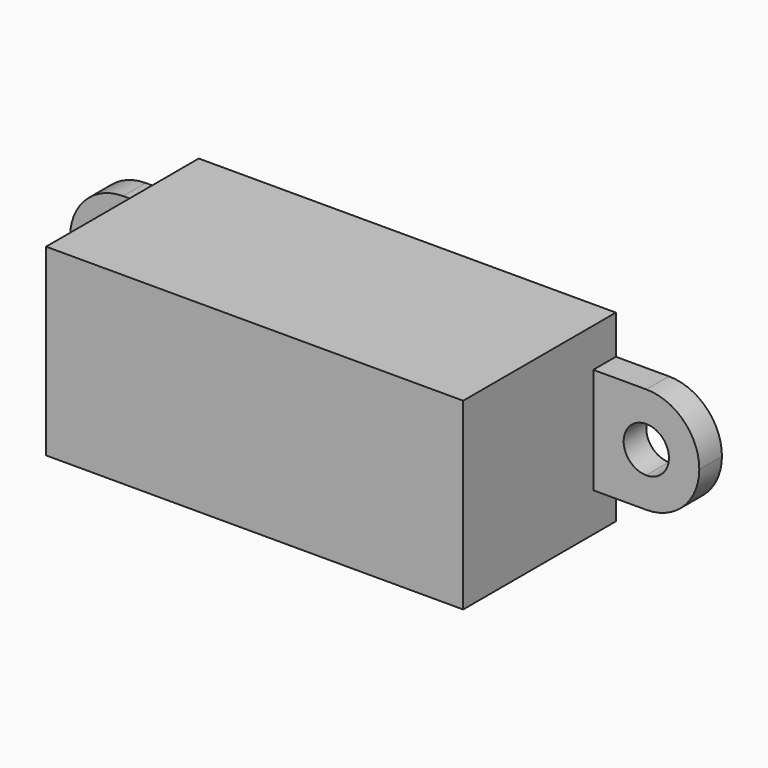
from build123d import *

# Parameters (mm, degrees)
F1_DEPTH = 13.5
F2_DEPTH = 2
F3_R     = 3.74999
F4_DEPTH = 2
F5_R     = 3.74999


# Not quite as in the source:
# - a fillet or chamfer is up to 0.001 mm smaller than in the source, because OpenCascade refuses the exact size
# - a feature names something its author has since deleted; it is built from what else it names


with BuildPart() as f1:
    # F0 (on Front) → F1 (new body)
    with BuildSketch(Plane.XZ):
        Polygon((2.2300408515, 13), (-27.2699591485, 13), (-27.2699591485, 10.2540537994), (-27.2699591485, 2.7540537994), (-27.2699591485, 0), (2.2300408515, 0), (2.2300408515, 2.75), (2.2300408515, 10.25), align=None)
    extrude(amount=F1_DEPTH)

    # F0 (on Front) → F2 (join)
    with BuildSketch(Plane.XZ):
        with BuildLine():
            Line((-27.2699591485, 2.7540537994), (-27.2699591485, 10.2540537994))
            Line((-27.2699591485, 10.2540537994), (-31.0199591485, 10.2540537994))
            Line((-31.0199591485, 10.2540537994), (-31.0199591485, 8.1040537994))
            ThreePointArc((-31.0199591485, 8.1040537994), (-29.8885882986, 7.6354246493), (-29.4199591485, 6.5040537994))
            ThreePointArc((-29.4199591485, 6.5040537994), (-31.0199591485, 4.9040537994), (-32.6199591485, 6.5040537994))
            Line((-32.6199591485, 6.5040537994), (-34.7699591485, 6.5040537994))
            Line((-34.7699591485, 6.5040537994), (-34.7699591485, 2.7540537994))
            Line((-34.7699591485, 2.7540537994), (-27.2699591485, 2.7540537994))
        make_face()
        with BuildLine():
            Line((-31.0199591485, 8.1040537994), (-31.0199591485, 10.2540537994))
            Line((-31.0199591485, 10.2540537994), (-34.7699591485, 10.2540537994))
            Line((-34.7699591485, 10.2540537994), (-34.7699591485, 6.5040537994))
            Line((-34.7699591485, 6.5040537994), (-32.6199591485, 6.5040537994))
            ThreePointArc((-32.6199591485, 6.5040537994), (-32.1513299984, 7.6354246493), (-31.0199591485, 8.1040537994))
        make_face()
    extrude(amount=F2_DEPTH)

    # F3 (radius 3.75 in the source; OpenCascade refuses exactly that, so slightly less here)
    f3_edges = [f1.edges().sort_by_distance(p)[0] for p in [
        (-34.769959, -1, 10.254054),
        (-34.769959, -1, 2.754054),
    ]]
    fillet(f3_edges, radius=F3_R)

    # F0 (on Front) → F4 (join)
    with BuildSketch(Plane.XZ):
        with BuildLine():
            Line((9.7300408515, 10.25), (2.2300408515, 10.25))
            Line((2.2300408515, 10.25), (2.2300408515, 2.75))
            Line((2.2300408515, 2.75), (5.9800408515, 2.75))
            Line((5.9800408515, 2.75), (5.9800408515, 4.9))
            ThreePointArc((5.9800408515, 4.9), (4.8486700016, 7.6313708499), (7.5800408515, 6.5))
            Line((7.5800408515, 6.5), (9.7300408515, 6.5))
            Line((9.7300408515, 6.5), (9.7300408515, 10.25))
        make_face()
        with BuildLine():
            Line((5.9800408515, 4.9), (5.9800408515, 2.75))
            Line((5.9800408515, 2.75), (9.7300408515, 2.75))
            Line((9.7300408515, 2.75), (9.7300408515, 6.5))
            Line((9.7300408515, 6.5), (7.5800408515, 6.5))
            ThreePointArc((7.5800408515, 6.5), (7.1114117014, 5.3686291501), (5.9800408515, 4.9))
        make_face()
    extrude(amount=F4_DEPTH)

    # F5 (radius 3.75 in the source; OpenCascade refuses exactly that, so slightly less here)
    f5_edges = [f1.edges().sort_by_distance(p)[0] for p in [
        (9.730041, -1, 10.25),
        (9.730041, -1, 2.75),
    ]]
    fillet(f5_edges, radius=F5_R)


solid = f1.part
